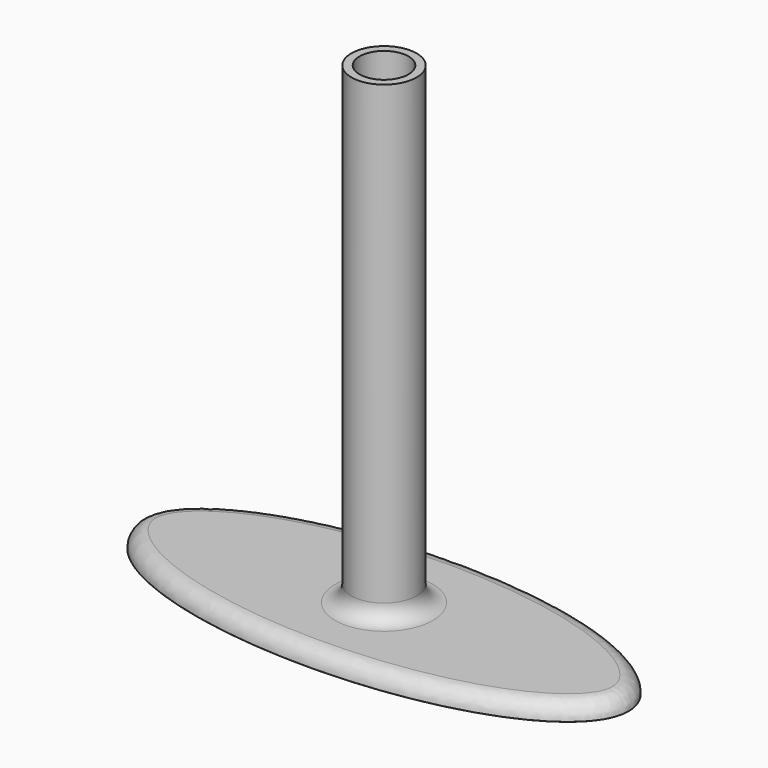
from build123d import *

# Parameters (mm, degrees)
F1_R     = 10
F2_DEPTH = 150
F3_T     = -2.5
F4_DEPTH = 5
F5_R     = 4.999


# Not quite as in the source:
# - a fillet or chamfer is up to 0.001 mm smaller than in the source, because OpenCascade refuses the exact size


with BuildPart() as f2:
    # F1 (on Top) → F2 (new body)
    with BuildSketch(Plane.XY):
        Circle(F1_R)
    extrude(amount=F2_DEPTH)

    # F3
    f3_openings = [f2.faces().sort_by_distance(p)[0] for p in [
        (0, 0, 150),
    ]]
    offset(amount=F3_T, openings=f3_openings)

    # F0 (on Top) → F4 (join)
    with BuildSketch(Plane.XY):
        with BuildLine():
            add(Edge.make_bspline(
                [(75, 0), (75, 51.9615242271), (-37.5, 25.9807621135), (-150, 0), (-37.5, -25.9807621135), (75, -51.9615242271), (75, 0)],
                knots=[0, 0, 0, 2.0943951024, 2.0943951024, 4.1887902048, 4.1887902048, 6.2831853072, 6.2831853072, 6.2831853072], degree=2, weights=[1, 0.5, 1, 0.5, 1, 0.5, 1]))
        make_face()
    extrude(amount=F4_DEPTH)

    # F5 (radius 5 in the source; OpenCascade refuses exactly that, so slightly less here)
    f5_edges = [f2.edges().sort_by_distance(p)[0] for p in [
        (-10, 0, 5),
        (-75, 9.6e-05, 5),
    ]]
    fillet(f5_edges, radius=F5_R)


solid = f2.part
